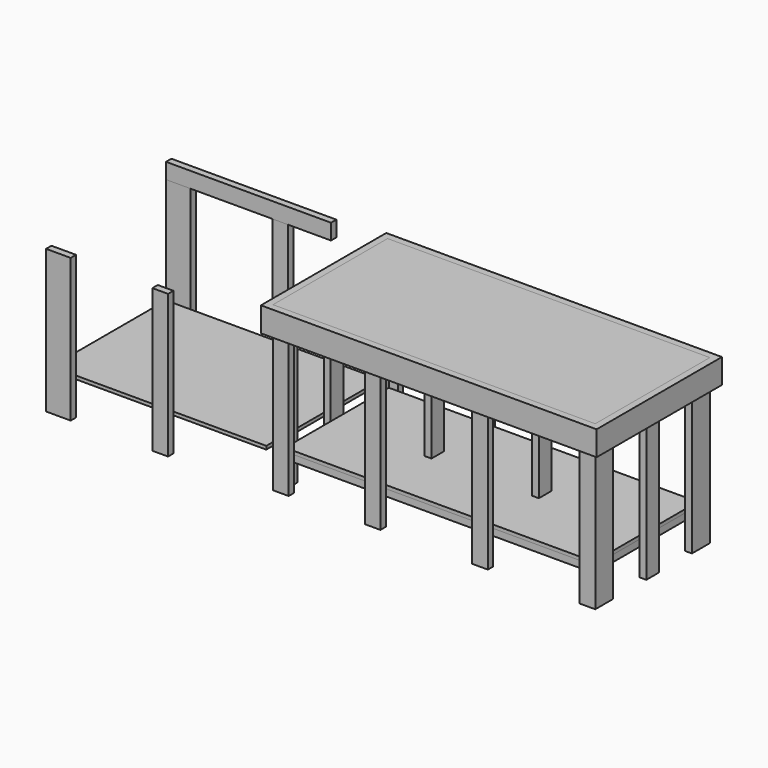
from build123d import *

# Parameters (mm, degrees)
F2_W           = 88.9
F2_H           = 38.1
F3_DEPTH       = 812.8
F2_W_2         = 38.1
F2_H_2         = 88.9
F4_DEPTH       = 152.4
F5_W           = 38.1
F5_H           = 660.4
F6_DEPTH       = 38.1
F7_W           = 1752.6
F7_H           = 736.6
F7_W_2         = 38.1
F7_H_2         = 88.9
F8_DEPTH       = 19.05
F7_W_3         = 1219.2
F7_H_3         = 812.8
F9_W           = 38.1
F9_H           = 736.6
F10_DEPTH      = 88.9
F9_W_2         = 936.1780285835
F9_H_2         = 38.1
F11_W          = 1828.8
F11_H          = 38.1
F12_DEPTH      = 25.4
F12_DEPTH_BACK = 114.3
F13_W          = 1828.8
F13_H          = 812.8
F14_DEPTH      = 19.05
F15_W          = 1828.8
F15_H          = 812.8
F16_DEPTH      = 6.35


# Not quite as in the source:
# - a feature names something its author has since deleted; it is built from what else it names


with BuildPart() as f3:
    # F2 (on Top) → F3 (new body)
    with BuildSketch(Plane.XY):
        with Locations((2432.05, 831.85)):
            Rectangle(F2_W, F2_H)
    extrude(amount=F3_DEPTH)


with BuildPart() as f3b:
    # F2 (on Top) → F3, piece 2 (new body)
    with BuildSketch(Plane.XY):
        with Locations((1822.45, 831.85)):
            Rectangle(F2_W, F2_H)
    extrude(amount=F3_DEPTH)


with BuildPart() as f3c:
    # F2 (on Top) → F3, piece 3 (new body)
    with BuildSketch(Plane.XY):
        with Locations((647.7, 869.95)):
            Rectangle(F2_W, F2_H)
    extrude(amount=F3_DEPTH)


with BuildPart() as f3d:
    # F2 (on Top) → F3, piece 4 (new body)
    with BuildSketch(Plane.XY):
        with Locations((1822.45, 57.15)):
            Rectangle(F2_W, F2_H)
    extrude(amount=F3_DEPTH)


with BuildPart() as f3e:
    # F2 (on Top) → F3, piece 5 (new body)
    with BuildSketch(Plane.XY):
        with Locations((647.7, 19.05)):
            Rectangle(F2_W, F2_H)
    extrude(amount=F3_DEPTH)


with BuildPart() as f3f:
    # F2 (on Top) → F3, piece 6 (new body)
    with BuildSketch(Plane.XY):
        with Locations((2432.05, 57.15)):
            Rectangle(F2_W, F2_H)
    extrude(amount=F3_DEPTH)


with BuildPart() as f3g:
    # F2 (on Top) → F3, piece 7 (new body)
    with BuildSketch(Plane.XY):
        with Locations((2457.45, 444.5)):
            Rectangle(F2_W_2, F2_H_2)
    extrude(amount=F3_DEPTH)


with BuildPart() as f3h:
    # F2 (on Top) → F3, piece 8 (new body)
    with BuildSketch(Plane.XY):
        with Locations((3067.05, 444.5)):
            Rectangle(F2_W_2, F2_H_2)
    extrude(amount=F3_DEPTH)


with BuildPart() as f3i:
    # F2 (on Top) → F3, piece 9 (new body)
    with BuildSketch(Plane.XY):
        with Locations((1847.85, 444.5)):
            Rectangle(F2_W_2, F2_H_2)
    extrude(amount=F3_DEPTH)


with BuildPart() as f3j:
    # F2 (on Top) → F3, piece 10 (new body)
    with BuildSketch(Plane.XY):
        with Locations((1276.35, 444.5)):
            Rectangle(F2_W_2, F2_H_2)
    extrude(amount=F3_DEPTH)


with BuildPart() as f3k:
    # F2 (on Top) → F3, piece 11 (new body)
    with BuildSketch(Plane.XY):
        Polygon((3048, 812.8), (3086.1, 812.8), (3086.1, 850.9), (2997.2, 850.9), (2997.2, 812.8), align=None)
        with Locations((3067.05, 768.35)):
            Rectangle(F2_W_2, F2_H_2)
    extrude(amount=F3_DEPTH)


with BuildPart() as f3l:
    # F2 (on Top) → F3, piece 12 (new body)
    with BuildSketch(Plane.XY):
        Polygon((1346.2, 812.8), (1346.2, 850.9), (1257.3, 850.9), (1257.3, 812.8), (1295.4, 812.8), align=None)
        with Locations((1276.35, 768.35)):
            Rectangle(F2_W_2, F2_H_2)
    extrude(amount=F3_DEPTH)


with BuildPart() as f3m:
    # F2 (on Top) → F3, piece 13 (new body)
    with BuildSketch(Plane.XY):
        Polygon((139.7, 889), (0, 889), (0, 850.9), (38.1, 850.9), (139.7, 850.9), align=None)
    extrude(amount=F3_DEPTH)


with BuildPart() as f3n:
    # F2 (on Top) → F3, piece 14 (new body)
    with BuildSketch(Plane.XY):
        Polygon((38.1, 38.1), (0, 38.1), (0, 0), (139.7, 0), (139.7, 38.1), align=None)
    extrude(amount=F3_DEPTH)


with BuildPart() as f3o:
    # F2 (on Top) → F3, piece 15 (new body)
    with BuildSketch(Plane.XY):
        Polygon((3086.1, 38.1), (3086.1, 76.2), (3048, 76.2), (2997.2, 76.2), (2997.2, 38.1), align=None)
        with Locations((3067.05, 120.65)):
            Rectangle(F2_W_2, F2_H_2)
    extrude(amount=F3_DEPTH)


with BuildPart() as f3p:
    # F2 (on Top) → F3, piece 16 (new body)
    with BuildSketch(Plane.XY):
        with Locations((1276.35, 120.65)):
            Rectangle(F2_W_2, F2_H_2)
        Polygon((1295.4, 76.2), (1257.3, 76.2), (1257.3, 38.1), (1346.2, 38.1), (1346.2, 76.2), align=None)
    extrude(amount=F3_DEPTH)


with BuildPart() as f4:
    # F2 (on Top) → F4 (new body)
    with BuildSketch(Plane.XY):
        with Locations((19.05, 444.5)):
            Rectangle(F2_W_2, F2_H_2)
    extrude(amount=F4_DEPTH)


with BuildPart() as f4b:
    # F2 (on Top) → F4, piece 2 (new body)
    with BuildSketch(Plane.XY):
        with Locations((647.7, 444.5)):
            Rectangle(F2_W_2, F2_H_2)
    extrude(amount=F4_DEPTH)


with BuildPart() as f4c:
    # F2 (on Top) → F4, piece 3 (new body)
    with BuildSketch(Plane.XY):
        with Locations((19.05, 806.45)):
            Rectangle(F2_W_2, F2_H_2)
    extrude(amount=F4_DEPTH)


with BuildPart() as f4d:
    # F2 (on Top) → F4, piece 4 (new body)
    with BuildSketch(Plane.XY):
        with Locations((19.05, 82.55)):
            Rectangle(F2_W_2, F2_H_2)
    extrude(amount=F4_DEPTH)


with BuildPart() as f6:
    # F5 (on offset) → F6 (new body)
    with BuildSketch(Plane.XY.offset(152.4)):
        Polygon((3048, 812.8), (1295.4, 812.8), (1295.4, 774.7), (1333.5, 774.7), (1790.7, 774.7), (1828.8, 774.7), (2400.3, 774.7), (2438.4, 774.7), (3009.9, 774.7), (3048, 774.7), align=None)
        with Locations((1314.45, 444.5)):
            Rectangle(F5_W, F5_H)
        with Locations((3028.95, 444.5)):
            Rectangle(F5_W, F5_H)
        Polygon((1333.5, 114.3), (1295.4, 114.3), (1295.4, 76.2), (3048, 76.2), (3048, 114.3), (3009.9, 114.3), (2438.4, 114.3), (2400.3, 114.3), (1828.8, 114.3), (1790.7, 114.3), align=None)
        with Locations((1809.75, 444.5)):
            Rectangle(F5_W, F5_H)
        with Locations((2419.35, 444.5)):
            Rectangle(F5_W, F5_H)
    extrude(amount=F6_DEPTH)


with BuildPart() as f8:
    # F7 (on face) → F8 (new body)
    with BuildSketch(Plane.XY.offset(190.5)):
        with Locations((2171.7, 444.5)):
            Rectangle(F7_W, F7_H)
        with Locations((1847.85, 444.5)):
            Rectangle(F7_W_2, F7_H_2, mode=Mode.SUBTRACT)
        with Locations((2457.45, 444.5)):
            Rectangle(F7_W_2, F7_H_2, mode=Mode.SUBTRACT)
    extrude(amount=F8_DEPTH)


with BuildPart() as f8b:
    # F7 (on face) → F8, piece 2 (new body)
    with BuildSketch(Plane.XY.offset(190.5)):
        with Locations((609.6, 444.5)):
            Rectangle(F7_W_3, F7_H_3)
    extrude(amount=F8_DEPTH)


with BuildPart() as f10:
    # F9 (on face) → F10 (new body)
    with BuildSketch(Plane.XY.offset(812.8)):
        Polygon((3048, 850.9), (1295.4, 850.9), (1295.4, 812.8), (1543.05, 812.8), (1581.15, 812.8), (1828.8, 812.8), (1866.9, 812.8), (2133.6, 812.8), (2171.7, 812.8), (2438.4, 812.8), (2476.5, 812.8), (2743.2, 812.8), (2781.3, 812.8), (3048, 812.8), align=None)
        Polygon((1295.4, 812.8), (1295.4, 850.9), (1257.3, 850.9), (1257.3, 38.1), (1295.4, 38.1), (1295.4, 76.2), align=None)
        Polygon((3086.1, 850.9), (3048, 850.9), (3048, 812.8), (3048, 76.2), (3048, 38.1), (3086.1, 38.1), align=None)
        Polygon((1543.05, 76.2), (1295.4, 76.2), (1295.4, 38.1), (3048, 38.1), (3048, 76.2), (2781.3, 76.2), (2743.2, 76.2), (2476.5, 76.2), (2438.4, 76.2), (2171.7, 76.2), (2133.6, 76.2), (1866.9, 76.2), (1828.8, 76.2), (1581.15, 76.2), align=None)
        with Locations((1562.1, 444.5)):
            Rectangle(F9_W, F9_H)
        with Locations((1847.85, 444.5)):
            Rectangle(F9_W, F9_H)
        with Locations((2152.65, 444.5)):
            Rectangle(F9_W, F9_H)
        with Locations((2457.45, 444.5)):
            Rectangle(F9_W, F9_H)
        with Locations((2762.25, 444.5)):
            Rectangle(F9_W, F9_H)
    extrude(amount=F10_DEPTH)

    # F13 (on face) → F14 (join)
    with BuildSketch(Plane.XY.offset(901.7)):
        with Locations((2171.7, 444.5)):
            Rectangle(F13_W, F13_H)
    extrude(amount=F14_DEPTH)

    # F15 (on face) → F16 (join)
    with BuildSketch(Plane.XY.offset(920.75)):
        with Locations((2171.7, 444.5)):
            Rectangle(F15_W, F15_H)
    extrude(amount=F16_DEPTH)


with BuildPart() as f10b:
    # F9 (on face) → F10, piece 2 (new body)
    with BuildSketch(Plane.XY.offset(812.8)):
        with Locations((468.0890142918, 869.95)):
            Rectangle(F9_W_2, F9_H_2)
    extrude(amount=F10_DEPTH)


with BuildPart() as f12:
    # F11 (on face) → F12 (new body, two sides)
    with BuildSketch(Plane.XY.offset(901.7)) as f12_sk:
        with Locations((2171.7, 869.95)):
            Rectangle(F11_W, F11_H)
        Polygon((3124.2, 889), (3086.1, 889), (3086.1, 850.9), (3086.1, 38.1), (3086.1, 0), (3124.2, 0), align=None)
        Polygon((1257.3, 850.9), (1257.3, 889), (1219.2, 889), (1219.2, 0), (1257.3, 0), (1257.3, 38.1), align=None)
        with Locations((2171.7, 19.05)):
            Rectangle(F11_W, F11_H)
    extrude(amount=F12_DEPTH)
    extrude(f12_sk.sketch, amount=-F12_DEPTH_BACK)


solid = Compound([f3.part, f3b.part, f3c.part, f3d.part, f3e.part, f3f.part, f3g.part, f3h.part, f3i.part, f3j.part, f3k.part, f3l.part, f3m.part, f3n.part, f3o.part, f3p.part, f4.part, f4b.part, f4c.part, f4d.part, f6.part, f8.part, f8b.part, f10.part, f10b.part, f12.part])
